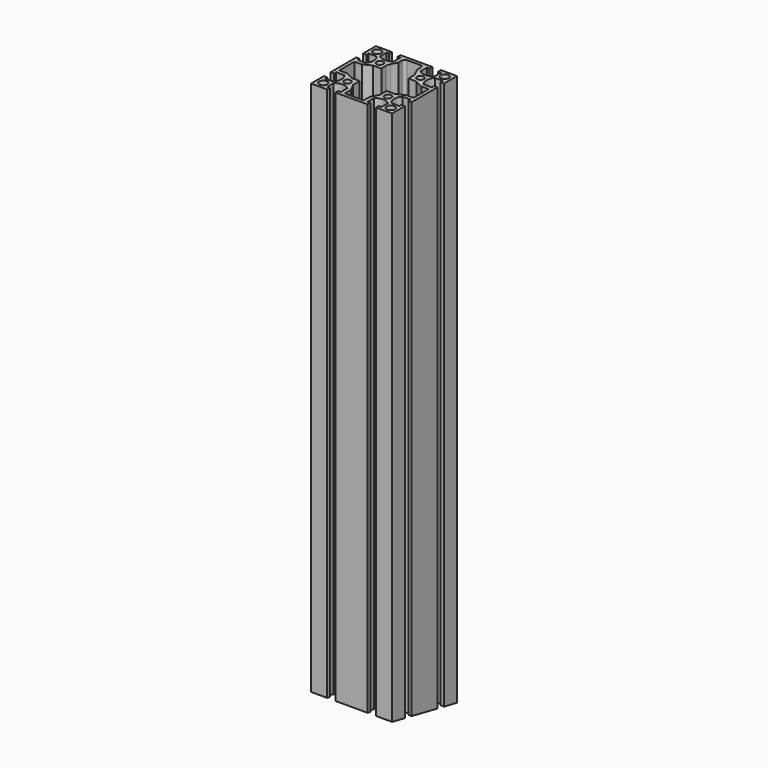
from build123d import *

# Parameters (mm, degrees)
F0_R          = 3
F0_R_2        = 2.5
F1_DEPTH      = 408.599
F2_R          = 2
F3_R          = 7
F5_DEPTH      = 30
F5_DEPTH_BACK = 30


# Not quite as in the source:
# - a feature names something its author has since deleted; it is built from what else it names


with BuildPart() as f1:
    # F0 (on Top) → F1 (new body)
    with BuildSketch(Plane.XY):
        with BuildLine():
            Line((18.15, -30), (30, -30))
            Line((30, -30), (30, -18.15))
            Line((30, -18.15), (27.5, -18.15))
            Line((27.5, -18.15), (27.5, -20.15))
            Line((27.5, -20.15), (21.5477069044, -20.15))
            ThreePointArc((21.5477069044, -20.15), (19.5, -15), (21.5477069044, -9.85))
            Line((21.5477069044, -9.85), (27.5, -9.85))
            Line((27.5, -9.85), (27.5, -11.85))
            Line((27.5, -11.85), (30, -11.85))
            Line((30, -11.85), (30, 11.85))
            Line((30, 11.85), (27.5, 11.85))
            Line((27.5, 11.85), (27.5, 9.85))
            Line((27.5, 9.85), (21.5477069044, 9.85))
            ThreePointArc((21.5477069044, 9.85), (19.5, 15), (21.5477069044, 20.15))
            Line((21.5477069044, 20.15), (27.5, 20.15))
            Line((27.5, 20.15), (27.5, 18.15))
            Line((27.5, 18.15), (30, 18.15))
            Line((30, 18.15), (30, 30))
            Line((30, 30), (18.15, 30))
            Line((18.15, 30), (18.15, 27.5))
            Line((18.15, 27.5), (20.15, 27.5))
            Line((20.15, 27.5), (20.15, 21.5477069044))
            ThreePointArc((20.15, 21.5477069044), (15, 19.5), (9.85, 21.5477069044))
            Line((9.85, 21.5477069044), (9.85, 27.5))
            Line((9.85, 27.5), (11.85, 27.5))
            Line((11.85, 27.5), (11.85, 30))
            Line((11.85, 30), (-11.85, 30))
            Line((-11.85, 30), (-11.85, 27.5))
            Line((-11.85, 27.5), (-9.85, 27.5))
            Line((-9.85, 27.5), (-9.85, 21.5477069044))
            ThreePointArc((-9.85, 21.5477069044), (-15, 19.5), (-20.15, 21.5477069044))
            Line((-20.15, 21.5477069044), (-20.15, 27.5))
            Line((-20.15, 27.5), (-18.15, 27.5))
            Line((-18.15, 27.5), (-18.15, 30))
            Line((-18.15, 30), (-30, 30))
            Line((-30, 30), (-30, 18.15))
            Line((-30, 18.15), (-27.5, 18.15))
            Line((-27.5, 18.15), (-27.5, 20.15))
            Line((-27.5, 20.15), (-21.5477069044, 20.15))
            ThreePointArc((-21.5477069044, 20.15), (-19.5, 15), (-21.5477069044, 9.85))
            Line((-21.5477069044, 9.85), (-27.5, 9.85))
            Line((-27.5, 9.85), (-27.5, 11.85))
            Line((-27.5, 11.85), (-30, 11.85))
            Line((-30, 11.85), (-30, -11.85))
            Line((-30, -11.85), (-27.5, -11.85))
            Line((-27.5, -11.85), (-27.5, -9.85))
            Line((-27.5, -9.85), (-21.5477069044, -9.85))
            ThreePointArc((-21.5477069044, -9.85), (-19.5, -15), (-21.5477069044, -20.15))
            Line((-21.5477069044, -20.15), (-27.5, -20.15))
            Line((-27.5, -20.15), (-27.5, -18.15))
            Line((-27.5, -18.15), (-30, -18.15))
            Line((-30, -18.15), (-30, -30))
            Line((-30, -30), (-18.15, -30))
            Line((-18.15, -30), (-18.15, -27.5))
            Line((-18.15, -27.5), (-20.15, -27.5))
            Line((-20.15, -27.5), (-20.15, -21.5477069044))
            ThreePointArc((-20.15, -21.5477069044), (-15, -19.5), (-9.85, -21.5477069044))
            Line((-9.85, -21.5477069044), (-9.85, -27.5))
            Line((-9.85, -27.5), (-11.85, -27.5))
            Line((-11.85, -27.5), (-11.85, -30))
            Line((-11.85, -30), (11.85, -30))
            Line((11.85, -30), (11.85, -27.5))
            Line((11.85, -27.5), (9.85, -27.5))
            Line((9.85, -27.5), (9.85, -21.5477069044))
            ThreePointArc((9.85, -21.5477069044), (15, -19.5), (20.15, -21.5477069044))
            Line((20.15, -21.5477069044), (20.15, -27.5))
            Line((20.15, -27.5), (18.15, -27.5))
            Line((18.15, -27.5), (18.15, -30))
        make_face()
        with Locations((-25, -25)):
            Circle(F0_R, mode=Mode.SUBTRACT)
        with Locations((-15, -15)):
            Circle(F0_R_2, mode=Mode.SUBTRACT)
        with Locations((25, -25)):
            Circle(F0_R, mode=Mode.SUBTRACT)
        with Locations((15, -15)):
            Circle(F0_R_2, mode=Mode.SUBTRACT)
        with Locations((-25, 25)):
            Circle(F0_R, mode=Mode.SUBTRACT)
        with Locations((-15, 15)):
            Circle(F0_R_2, mode=Mode.SUBTRACT)
        Polygon((-7, 22), (-7, 27.5), (0, 27.5), (7, 27.5), (7, 22), (10, 16), (10, 10), (16, 10), (22, 7), (27.5, 7), (27.5, 0), (27.5, -7), (22, -7), (16, -10), (10, -10), (10, -16), (7, -22), (7, -27.5), (0, -27.5), (-7, -27.5), (-7, -22), (-10, -16), (-10, -10), (-16, -10), (-22, -7), (-27.5, -7), (-27.5, 0), (-27.5, 7), (-22, 7), (-16, 10), (-10, 10), (-10, 16), align=None, mode=Mode.SUBTRACT)
        with Locations((15, 15)):
            Circle(F0_R_2, mode=Mode.SUBTRACT)
        with Locations((25, 25)):
            Circle(F0_R, mode=Mode.SUBTRACT)
    extrude(amount=F1_DEPTH)

    # F2
    f2_edges = [f1.edges().sort_by_distance(p)[0] for p in [
        (-7, 27.5, 204.2995),
        (7, 27.5, 204.2995),
    ]]
    fillet(f2_edges, radius=F2_R)

    # F3
    f3_edges = [f1.edges().sort_by_distance(p)[0] for p in [
        (-10, 16, 204.2995),
        (10, 16, 204.2995),
    ]]
    fillet(f3_edges, radius=F3_R)

    # F4 (on Right) → F5 (cut, two sides)
    with BuildSketch(Plane.YZ) as f5_sk:
        Polygon((-164.2855995683, 38.6458085579), (-188.5911429791, -83.5464097089), (5.6944565892, -122.1922182668), (30, 0), align=None)
    extrude(amount=F5_DEPTH, mode=Mode.SUBTRACT)
    extrude(f5_sk.sketch, amount=-F5_DEPTH_BACK, mode=Mode.SUBTRACT)


solid = f1.part
